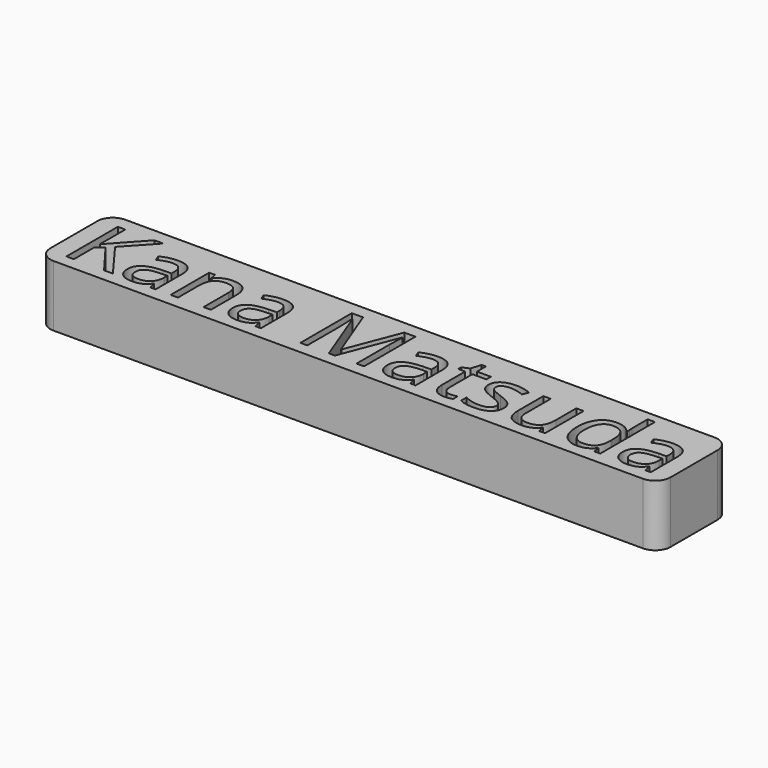
from build123d import *

# Parameters (mm, degrees)
F2_DEPTH     = 25.4
F0_TEXT_SIZE = 37.2943364912
F3_DEPTH     = 19.05


# Not quite as in the source:
# - Text() gives the source's letters only with a copy of the font that has no kerning and outlines rounded to 1/6400 em; it was checked with that copy


with BuildPart() as f2:
    # F1 (on Top) → F2 (new body)
    with BuildSketch(Plane.XY):
        with BuildLine():
            Line((195.4707013607, 31.9748073816), (-48.8374823868, 31.9748073816))
            ThreePointArc((-48.8374823868, 31.9748073816), (-53.3276104474, 30.1149354422), (-55.1874823868, 25.6248073816))
            Line((-55.1874823868, 25.6248073816), (-55.1874823868, 1.2347033083))
            ThreePointArc((-55.1874823868, 1.2347033083), (-53.3276104474, -3.2554247522), (-48.8374823868, -5.1152966917))
            Line((-48.8374823868, -5.1152966917), (195.4707013607, -5.1152966917))
            ThreePointArc((195.4707013607, -5.1152966917), (199.9608294212, -3.2554247522), (201.8207013607, 1.2347033083))
            Line((201.8207013607, 1.2347033083), (201.8207013607, 25.6248073816))
            ThreePointArc((201.8207013607, 25.6248073816), (199.9608294212, 30.1149354422), (195.4707013607, 31.9748073816))
        make_face()
    extrude(amount=-F2_DEPTH)

    # F0 (on Top) → F3 (cut)
    with BuildSketch(Plane.XY):
        with Locations((-51.1933006346, 0)):
            Text('Kana Matsuda', F0_TEXT_SIZE, font='Open Sans', text_align=(TextAlign.LEFT, TextAlign.BOTTOM))
    extrude(amount=-F3_DEPTH, mode=Mode.SUBTRACT)


solid = f2.part
